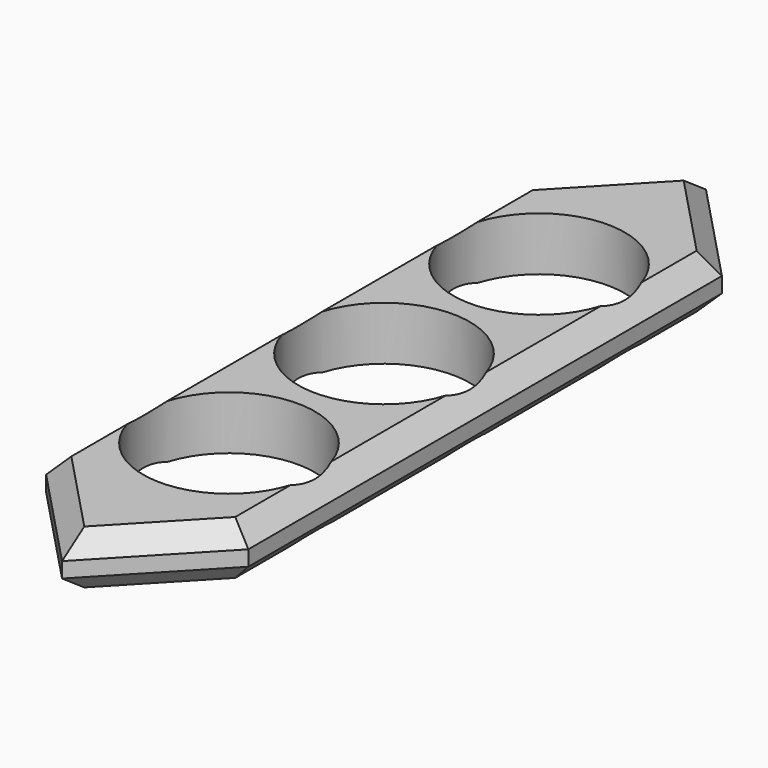
from build123d import *

# Parameters (mm, degrees)
F0_R        = 11.2
F1_DEPTH    = 7
F2_T1_DEPTH = 32.0222283479
F2_T3_DEPTH = 32.0222283479
F2_T5_DEPTH = 90.1351514377
F2_T7_DEPTH = 32.0222283479
F2_T9_DEPTH = 32.0222283479
F3_T1_DEPTH = 32.0222283479
F3_T3_DEPTH = 32.0222283479
F3_T5_DEPTH = 90.1351514377
F3_T7_DEPTH = 32.0222283479
F3_T9_DEPTH = 32.0222283479


# Not quite as in the source:
# - a fillet or chamfer that OpenCascade refuses, or shapes differently, is made with other operations: its cross-section is extruded or revolved along the edge and cut away or added


with BuildPart() as f1:
    # F0 (on Top) → F1 (new body)
    with BuildSketch(Plane.XY):
        with BuildLine():
            ThreePointArc((-13.2, 0), (0, 13.2), (13.2, 0))
            Line((13.2, 0), (13.2, 38.6383682489))
            Line((13.2, 38.6383682489), (0, 52.53123492))
            Line((0, 52.53123492), (-13.2, 38.6383682489))
            Line((-13.2, 38.6383682489), (-13.2, 0))
        make_face()
        with Locations((0, 25.2957735211)):
            Circle(F0_R, mode=Mode.SUBTRACT)
        with BuildLine():
            Line((13.2, -38.6383682489), (13.2, 0))
            ThreePointArc((13.2, 0), (0, -13.2), (-13.2, 0))
            Line((-13.2, 0), (-13.2, -38.6383682489))
            Line((-13.2, -38.6383682489), (0, -52.53123492))
            Line((0, -52.53123492), (13.2, -38.6383682489))
        make_face()
        with Locations((0, -25.2957735211)):
            Circle(F0_R, mode=Mode.SUBTRACT)
        with BuildLine():
            ThreePointArc((-13.2, 0), (0, -13.2), (13.2, 0))
            ThreePointArc((13.2, 0), (0, 13.2), (-13.2, 0))
        make_face()
        Circle(F0_R, mode=Mode.SUBTRACT)
    extrude(amount=F1_DEPTH)

    # F2: chamfer of 2.5 on 6 edges, made by hand

    # F2_s2 → F2_t1 (cut)
    with BuildSketch(Plane(origin=(-30.6597100359, -32.269035129, 0), x_dir=(0, 0, 1), z_dir=(0.6887981906, 0.7249531383, 0))):
        Polygon((4.5, 36.1834195615), (7, 33.6834195615), (7, 36.1834195615), align=None)
    extrude(amount=F2_T1_DEPTH, mode=Mode.SUBTRACT)

    # F2_s4 → F2_t3 (cut)
    with BuildSketch(Plane(origin=(8.6028570917, -9.0544201944, 0), x_dir=(0, 0, 1), z_dir=(0.6887981906, -0.7249531383, 0))):
        Polygon((4.5, 36.1834195615), (7, 33.6834195615), (7, 36.1834195615), align=None)
    extrude(amount=F2_T3_DEPTH, mode=Mode.SUBTRACT)

    # F2_s6 → F2_t5 (cut)
    with BuildSketch(Plane.XZ.offset(-45.0675757189)):
        Polygon((13.2, 4.5), (10.7, 7), (13.2, 7), align=None)
        Polygon((-13.2, 4.5), (-10.7, 7), (-13.2, 7), align=None)
    extrude(amount=F2_T5_DEPTH, mode=Mode.SUBTRACT)

    # F2_s8 → F2_t7 (cut)
    with BuildSketch(Plane(origin=(30.6597100359, 32.269035129, 0), x_dir=(0, 0, 1), z_dir=(-0.6887981906, -0.7249531383, 0))):
        Polygon((4.5, 36.1834195615), (7, 33.6834195615), (7, 36.1834195615), align=None)
    extrude(amount=F2_T7_DEPTH, mode=Mode.SUBTRACT)

    # F2_s10 → F2_t9 (cut)
    with BuildSketch(Plane(origin=(-8.6028570917, 9.0544201944, 0), x_dir=(0, 0, 1), z_dir=(-0.6887981906, 0.7249531383, 0))):
        Polygon((4.5, 36.1834195615), (7, 33.6834195615), (7, 36.1834195615), align=None)
    extrude(amount=F2_T9_DEPTH, mode=Mode.SUBTRACT)

    # F3: chamfer of 2.5 on 6 edges, made by hand

    # F3_s2 → F3_t1 (cut)
    with BuildSketch(Plane(origin=(8.6028570917, -9.0544201944, 0), x_dir=(0, 0, 1), z_dir=(0.6887981906, -0.7249531383, 0))):
        Polygon((0, 33.6834195615), (2.5, 36.1834195615), (0, 36.1834195615), align=None)
    extrude(amount=F3_T1_DEPTH, mode=Mode.SUBTRACT)

    # F3_s4 → F3_t3 (cut)
    with BuildSketch(Plane(origin=(-30.6597100359, -32.269035129, 0), x_dir=(0, 0, 1), z_dir=(0.6887981906, 0.7249531383, 0))):
        Polygon((0, 33.6834195615), (2.5, 36.1834195615), (0, 36.1834195615), align=None)
    extrude(amount=F3_T3_DEPTH, mode=Mode.SUBTRACT)

    # F3_s6 → F3_t5 (cut)
    with BuildSketch(Plane.XZ.offset(-45.0675757189)):
        Polygon((10.7, 0), (13.2, 2.5), (13.2, 0), align=None)
        Polygon((-10.7, 0), (-13.2, 2.5), (-13.2, 0), align=None)
    extrude(amount=F3_T5_DEPTH, mode=Mode.SUBTRACT)

    # F3_s8 → F3_t7 (cut)
    with BuildSketch(Plane(origin=(30.6597100359, 32.269035129, 0), x_dir=(0, 0, 1), z_dir=(-0.6887981906, -0.7249531383, 0))):
        Polygon((0, 33.6834195615), (2.5, 36.1834195615), (0, 36.1834195615), align=None)
    extrude(amount=F3_T7_DEPTH, mode=Mode.SUBTRACT)

    # F3_s10 → F3_t9 (cut)
    with BuildSketch(Plane(origin=(-8.6028570917, 9.0544201944, 0), x_dir=(0, 0, 1), z_dir=(-0.6887981906, 0.7249531383, 0))):
        Polygon((2.5, 36.1834195615), (0, 33.6834195615), (0, 36.1834195615), align=None)
    extrude(amount=F3_T9_DEPTH, mode=Mode.SUBTRACT)


solid = f1.part
